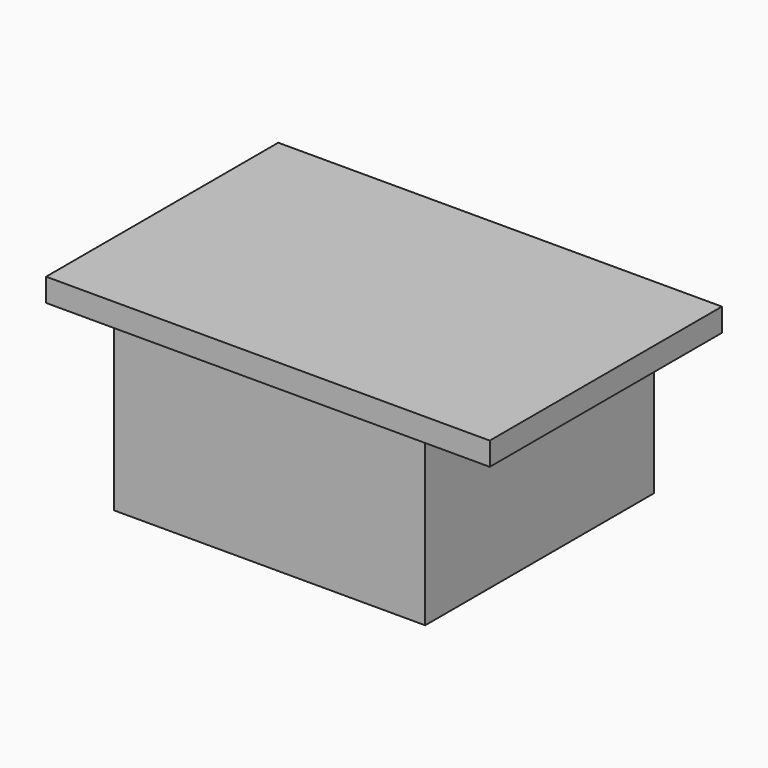
from build123d import *

# Parameters (mm, degrees)
F1_DEPTH      = 334.9625
F1_DEPTH_BACK = 334.9625
F2_W          = 100.0125
F2_H          = 431.8
F3_DEPTH      = 244.475


# Not quite as in the source:
# - a length typed as a fraction of an inch, garbled in the dataset ("3 / 203.2 mm" for 3/8 in), is restored


with BuildPart() as f1:
    # F0 (on Right) → F1 (new body, two sides)
    with BuildSketch(Plane.YZ) as f1_sk:
        Polygon((219.075, 127), (-219.075, 127), (-219.075, 92.075), (-215.9, 92.075), (-215.9, -152.4), (215.9, -152.4), (215.9, 92.075), (219.075, 92.075), align=None)
    extrude(amount=F1_DEPTH)
    extrude(f1_sk.sketch, amount=-F1_DEPTH_BACK)

    # F2 (on face) → F3 (cut, through all)
    with BuildSketch(Plane(origin=(0, 0, -152.4), x_dir=(1, 0, 0), z_dir=(0, 0, -1))):
        with Locations((-284.95625, 0)):
            Rectangle(F2_W, F2_H)
        with Locations((284.95625, 0)):
            Rectangle(F2_W, F2_H)
    extrude(amount=-F3_DEPTH, mode=Mode.SUBTRACT)


solid = f1.part
